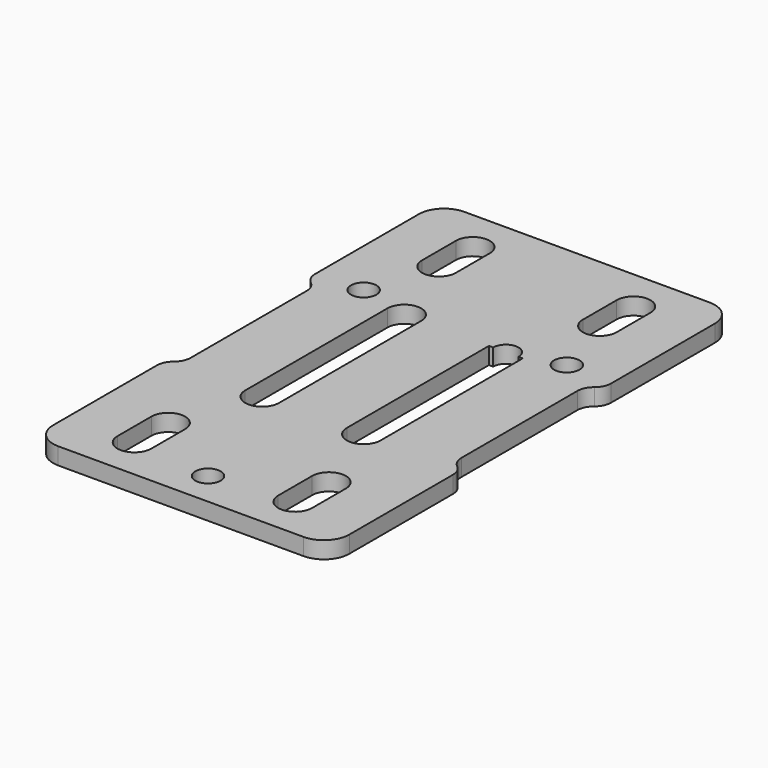
from build123d import *

# Parameters (mm, degrees)
F0_R        = 1.5
F1_DEPTH    = 2
F2_R        = 3
F3_W        = 4
F3_H        = 5
F3_W_2      = 1.5
F3_H_2      = 21
F4_DEPTH    = 2.001
F5_R        = 2
F5_R_2      = 1.5
F6_DEPTH    = 2.001
F7_T1_DEPTH = 2
F8_R        = 2


# Not quite as in the source:
# - a fillet or chamfer that OpenCascade refuses, or shapes differently, is made with other operations: its cross-section is extruded or revolved along the edge and cut away or added


with BuildPart() as f1:
    # F0 (on Top) → F1 (new body)
    with BuildSketch(Plane.XY):
        Polygon((-17.5, 17.5), (-17.5, -17.5), (-17.5, -30), (17.5, -30), (17.5, -17.5), (17.5, 17.5), (17.5, 30), (-17.5, 30), align=None)
        with Locations((0, -26)):
            Circle(F0_R, mode=Mode.SUBTRACT)
        with Locations((-12, 12)):
            Circle(F0_R, mode=Mode.SUBTRACT)
        with Locations((12, 12)):
            Circle(F0_R, mode=Mode.SUBTRACT)
    extrude(amount=F1_DEPTH)

    # F2
    f2_edges = [f1.edges().sort_by_distance(p)[0] for p in [
        (-17.5, -30, 1),
        (17.5, -30, 1),
        (17.5, 30, 1),
        (-17.5, 30, 1),
    ]]
    fillet(f2_edges, radius=F2_R)

    # F3 (on face) → F4 (cut, through all)
    with BuildSketch(Plane.XY.offset(2)):
        with Locations((9.5, 22.5)):
            Rectangle(F3_W, F3_H)
        with Locations((9.5, -22.5)):
            Rectangle(F3_W, F3_H)
        with Locations((-9.5, -22.5)):
            Rectangle(F3_W, F3_H)
        with Locations((-9.5, 22.5)):
            Rectangle(F3_W, F3_H)
        with Locations((-16.75, 0)):
            Rectangle(F3_W_2, F3_H_2)
        with Locations((16.75, 0)):
            Rectangle(F3_W_2, F3_H_2)
        with Locations((-6, 0)):
            Rectangle(F3_W, F3_H_2)
        with Locations((6, 0)):
            Rectangle(F3_W, F3_H_2)
    extrude(amount=-F4_DEPTH, mode=Mode.SUBTRACT)

    # F5 (on face) → F6 (cut, through all)
    with BuildSketch(Plane.XY.offset(2)):
        with Locations((-9.5, 25)):
            Circle(F5_R)
        with Locations((9.5, 25)):
            Circle(F5_R)
        with Locations((9.5, -25)):
            Circle(F5_R)
        with Locations((-9.5, -25)):
            Circle(F5_R)
        with Locations((-9.5, -20)):
            Circle(F5_R)
        with Locations((9.5, -20)):
            Circle(F5_R)
        with Locations((6, -10.5)):
            Circle(F5_R)
        with Locations((-6, -10.5)):
            Circle(F5_R)
        with Locations((-6, 10.5)):
            Circle(F5_R)
        with Locations((6, 10.5)):
            Circle(F5_R_2)
        with Locations((9.5, 20)):
            Circle(F5_R)
        with Locations((-9.5, 20)):
            Circle(F5_R)
    extrude(amount=-F6_DEPTH, mode=Mode.SUBTRACT)

    # F7: fillet of radius 2 on 4 edges, made by hand

    # F7_s2 → F7_t1 (join)
    with BuildSketch(Plane.XY):
        with BuildLine():
            ThreePointArc((-17.5, -10.5), (-16.4188611699, -9.7882531983), (-16, -8.5635083269))
            Line((-16, -8.5635083269), (-16, -10.5))
            Line((-16, -10.5), (-17.5, -10.5))
        make_face()
        with BuildLine():
            ThreePointArc((-17.5, 10.5), (-16.4188611699, 9.7882531983), (-16, 8.5635083269))
            Line((-16, 8.5635083269), (-16, 10.5))
            Line((-16, 10.5), (-17.5, 10.5))
        make_face()
        with BuildLine():
            ThreePointArc((16, 8.5635083269), (16.4188611699, 9.7882531983), (17.5, 10.5))
            Line((17.5, 10.5), (16, 10.5))
            Line((16, 10.5), (16, 8.5635083269))
        make_face()
        with BuildLine():
            ThreePointArc((17.5, -10.5), (16.4188611699, -9.7882531983), (16, -8.5635083269))
            Line((16, -8.5635083269), (16, -10.5))
            Line((16, -10.5), (17.5, -10.5))
        make_face()
    extrude(amount=F7_T1_DEPTH)

    # F8
    f8_edges = [f1.edges().sort_by_distance(p)[0] for p in [
        (17.5, -10.5, 1),
        (17.5, 10.5, 1),
        (-17.5, -10.5, 1),
        (-17.5, 10.5, 1),
    ]]
    fillet(f8_edges, radius=F8_R)


solid = f1.part
